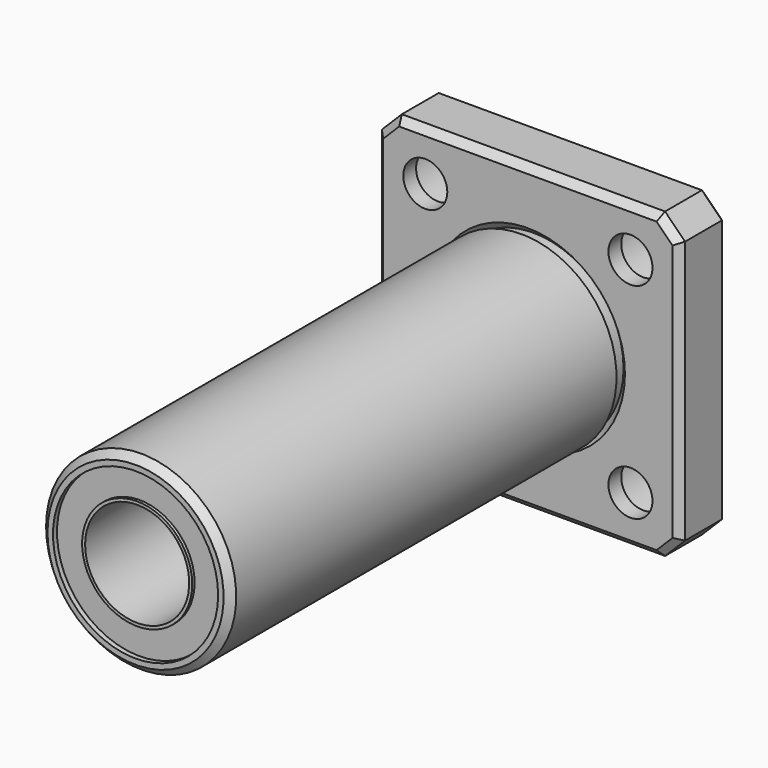
from build123d import *

# Parameters (mm, degrees)
F0_W           = 30.3
F0_H           = 30.3
F0_R           = 9
F1_DEPTH       = 6
F3_SIZE        = 2
F5_SIZE        = 0.7
F5_2_SIZE      = 0.7
F7_D           = 4.4
F7_CBORE_D     = 8
F7_CBORE_DEPTH = 4.4
F9_R           = 9
F9_R_2         = 5.5
F10_DEPTH      = 0.7
F9_R_3         = 5.2
F11_DEPTH      = 0.4
F12_DEPTH      = 55
F13_R          = 8.25
F13_R_2        = 5.5
F14_DEPTH      = 0.5
F13_R_3        = 5.2
F15_DEPTH      = 0.2


# Not quite as in the source:
# - two fillets or chamfers of one size are made in one step


with BuildPart() as f1:
    # F0 (on Front) → F1 (new body)
    with BuildSketch(Plane.XZ):
        Rectangle(F0_W, F0_H)
        Circle(F0_R, mode=Mode.SUBTRACT)
    extrude(amount=-F1_DEPTH)

    # F3
    f3_edges = [f1.edges().sort_by_distance(p)[0] for p in [
        (15.15, 3, 15.15),
        (-15.15, 3, 15.15),
        (15.15, 3, -15.15),
        (-15.15, 3, -15.15),
    ]]
    chamfer(f3_edges, length=F3_SIZE)

    # F5
    f5_edges = [f1.edges().sort_by_distance(p)[0] for p in [
        (9, 3, 0),
        (-9, 0, 0),
        (-9, 6, 0),
        (0, 0, 15.15),
        (-14.15, 0, 14.15),
        (-15.15, 0, 0),
        (-14.15, 0, -14.15),
        (0, 0, -15.15),
        (14.15, 0, -14.15),
        (15.15, 0, 0),
        (14.15, 0, 14.15),
        (15.15, 6, 0),
        (14.15, 6, 14.15),
        (0, 6, 15.15),
        (-14.15, 6, 14.15),
        (-15.15, 6, 0),
        (-14.15, 6, -14.15),
        (0, 6, -15.15),
        (14.15, 6, -14.15),
    ]]
    chamfer(f5_edges, length=F5_SIZE)

    # F7 (through all)
    with Locations(Plane(origin=(0, 6, 0), x_dir=(-1, 0, 0), z_dir=(0, 1, 0))):
        with Locations((-10.25, 10.25), (10.25, 10.25), (10.25, -10.25), (-10.25, -10.25)):
            CounterBoreHole(F7_D / 2, F7_CBORE_D / 2, F7_CBORE_DEPTH)


with BuildPart() as f4:
    # F2 (on Top) → F4 (revolve)
    with BuildSketch(Plane.XY):
        Polygon((0, -49), (0, 6), (-9, 6), (-9, -0.8), (-9.5, -0.8), (-9.5, -49), align=None)
    revolve(axis=Axis((0, 15.3594217002, 0), (0, -1, 0)))

    # F5#2
    f5_2_edges = [f4.edges().sort_by_distance(p)[0] for p in [
        (9.5, -49, 0),
    ]]
    chamfer(f5_2_edges, length=F5_2_SIZE)

    # F9 (on face) → F10 (cut)
    with BuildSketch(Plane(origin=(0, 6, 0), x_dir=(-1, 0, 0), z_dir=(0, 1, 0))):
        Circle(F9_R)
        Circle(F9_R_2, mode=Mode.SUBTRACT)
    extrude(amount=-F10_DEPTH, mode=Mode.SUBTRACT)

    # F9 (on face) → F11 (cut)
    with BuildSketch(Plane(origin=(0, 6, 0), x_dir=(-1, 0, 0), z_dir=(0, 1, 0))):
        Circle(F9_R_2)
        Circle(F9_R_3, mode=Mode.SUBTRACT)
    extrude(amount=-F11_DEPTH, mode=Mode.SUBTRACT)

    # F9 (on face) → F12 (cut, through all)
    with BuildSketch(Plane(origin=(0, 6, 0), x_dir=(-1, 0, 0), z_dir=(0, 1, 0))):
        Circle(F9_R_3)
    extrude(amount=-F12_DEPTH, mode=Mode.SUBTRACT)

    # F13 (on face) → F14 (cut)
    with BuildSketch(Plane.XZ.offset(49)):
        Circle(F13_R)
        Circle(F13_R_2, mode=Mode.SUBTRACT)
    extrude(amount=-F14_DEPTH, mode=Mode.SUBTRACT)

    # F13 (on face) → F15 (cut)
    with BuildSketch(Plane.XZ.offset(49)):
        Circle(F13_R_2)
        Circle(F13_R_3, mode=Mode.SUBTRACT)
    extrude(amount=-F15_DEPTH, mode=Mode.SUBTRACT)


solid = Compound([f1.part, f4.part])
